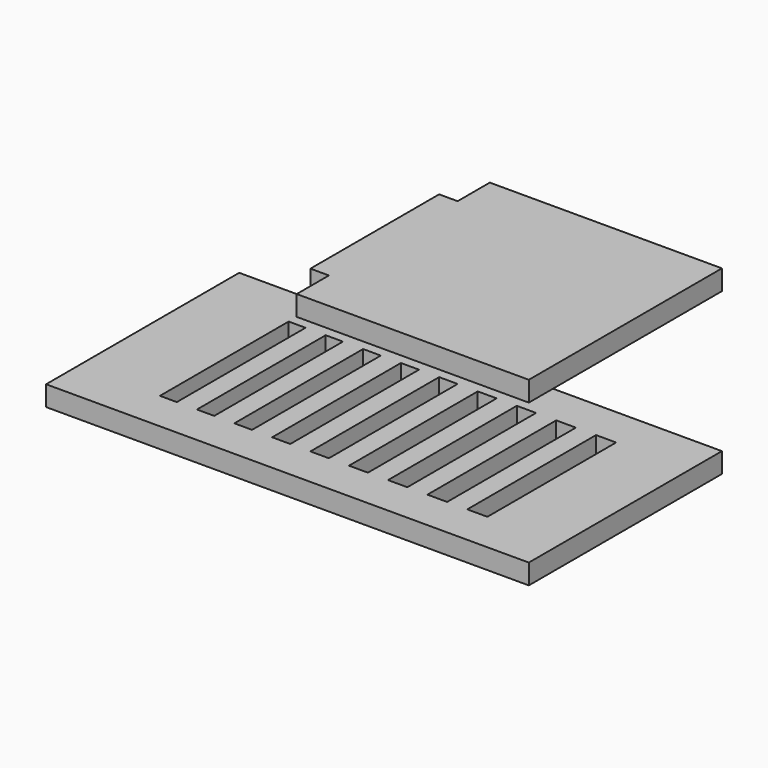
from build123d import *

# Parameters (mm, degrees)
F1_W     = 76.2
F1_H     = 38.1
F1_W_2   = 2.667
F1_H_2   = 25.4
F1_W_3   = 2.7305
F1_W_4   = 2.794
F1_W_5   = 2.8575
F1_W_6   = 2.921
F1_W_7   = 2.9845
F1_W_8   = 3.048
F1_W_9   = 3.1115
F1_W_10  = 3.175
F2_DEPTH = 3.175
F5_DEPTH = 3.175


# Not quite as in the source:
# - a variable given as a bare number and used for a length is read in inches; the dataset says mm whatever the document's units were


with BuildPart() as f2:
    # F1 (on Top) → F2 (new body)
    with BuildSketch(Plane.XY):
        Rectangle(F1_W, F1_H)
        with Locations((-23.876, 0)):
            Rectangle(F1_W_2, F1_H_2, mode=Mode.SUBTRACT)
        with Locations((-18.00225, 0)):
            Rectangle(F1_W_3, F1_H_2, mode=Mode.SUBTRACT)
        with Locations((-12.065, 0)):
            Rectangle(F1_W_4, F1_H_2, mode=Mode.SUBTRACT)
        with Locations((-6.06425, 0)):
            Rectangle(F1_W_5, F1_H_2, mode=Mode.SUBTRACT)
        Rectangle(F1_W_6, F1_H_2, mode=Mode.SUBTRACT)
        with Locations((6.12775, 0)):
            Rectangle(F1_W_7, F1_H_2, mode=Mode.SUBTRACT)
        with Locations((12.319, 0)):
            Rectangle(F1_W_8, F1_H_2, mode=Mode.SUBTRACT)
        with Locations((18.57375, 0)):
            Rectangle(F1_W_9, F1_H_2, mode=Mode.SUBTRACT)
        with Locations((24.892, 0)):
            Rectangle(F1_W_10, F1_H_2, mode=Mode.SUBTRACT)
    extrude(amount=F2_DEPTH)


with BuildPart() as f5:
    # F4 (on offset) → F5 (new body)
    with BuildSketch(Plane.XY.offset(25.4)):
        Polygon((1.4605, 12.7), (-1.4605, 12.7), (-1.4605, -12.7), (1.4605, -12.7), (1.4605, -19.05), (38.1, -19.05), (38.1, 19.05), (1.4605, 19.05), align=None)
    extrude(amount=F5_DEPTH)


solid = Compound([f2.part, f5.part])
